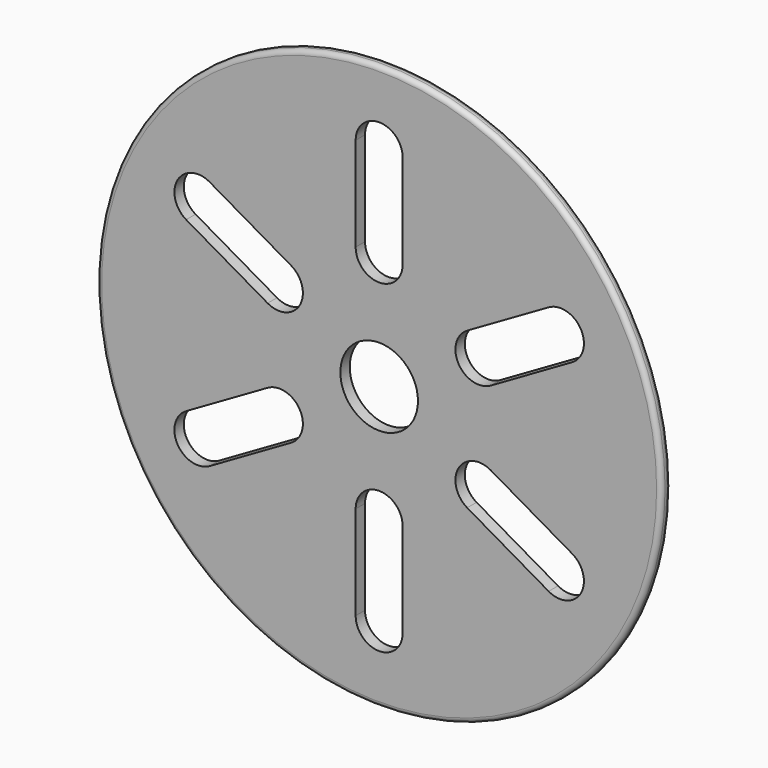
from build123d import *

# Parameters (mm, degrees)
F0_R     = 304.8
F0_R_2   = 41.91
F1_DEPTH = 12.7
F3_DEPTH = 12.701
F4_R     = 5.08


# Not quite as in the source:
# - a feature names something its author has since deleted; it is built from what else it names


with BuildPart() as f1:
    # F0 (on Front) → F1 (new body)
    with BuildSketch(Plane.XZ):
        Circle(F0_R)
        Circle(F0_R_2, mode=Mode.SUBTRACT)
    extrude(amount=F1_DEPTH)

    # F2 (on face) → F3 (cut, through all)
    with BuildSketch(Plane.XZ.offset(12.7)):
        with BuildLine():
            Line((-25.4, 226.06), (-25.4, 124.46))
            ThreePointArc((-25.4, 124.46), (0, 99.06), (25.4, 124.46))
            Line((25.4, 124.46), (25.4, 226.06))
            ThreePointArc((25.4, 226.06), (0, 251.46), (-25.4, 226.06))
        make_face()
        with BuildLine():
            Line((-183.0737027795, -135.0270452561), (-95.085521755, -84.2270452561))
            ThreePointArc((-95.085521755, -84.2270452561), (-85.7884764989, -49.53), (-120.485521755, -40.2329547439))
            Line((-120.485521755, -40.2329547439), (-208.4737027795, -91.0329547439))
            ThreePointArc((-208.4737027795, -91.0329547439), (-217.7707480356, -125.73), (-183.0737027795, -135.0270452561))
        make_face()
        with BuildLine():
            Line((-208.4737027795, 91.0329547439), (-120.485521755, 40.2329547439))
            ThreePointArc((-120.485521755, 40.2329547439), (-85.7884764989, 49.53), (-95.085521755, 84.2270452561))
            Line((-95.085521755, 84.2270452561), (-183.0737027795, 135.0270452561))
            ThreePointArc((-183.0737027795, 135.0270452561), (-217.7707480356, 125.73), (-208.4737027795, 91.0329547439))
        make_face()
        with BuildLine():
            Line((183.0737027795, 135.0270452561), (95.085521755, 84.2270452561))
            ThreePointArc((95.085521755, 84.2270452561), (85.7884764989, 49.53), (120.485521755, 40.2329547439))
            Line((120.485521755, 40.2329547439), (208.4737027795, 91.0329547439))
            ThreePointArc((208.4737027795, 91.0329547439), (217.7707480356, 125.73), (183.0737027795, 135.0270452561))
        make_face()
        with BuildLine():
            Line((208.4737027795, -91.0329547439), (120.485521755, -40.2329547439))
            ThreePointArc((120.485521755, -40.2329547439), (85.7884764989, -49.53), (95.085521755, -84.2270452561))
            Line((95.085521755, -84.2270452561), (183.0737027795, -135.0270452561))
            ThreePointArc((183.0737027795, -135.0270452561), (217.7707480356, -125.73), (208.4737027795, -91.0329547439))
        make_face()
        with BuildLine():
            Line((25.4, -226.06), (25.4, -124.46))
            ThreePointArc((25.4, -124.46), (0, -99.06), (-25.4, -124.46))
            Line((-25.4, -124.46), (-25.4, -226.06))
            ThreePointArc((-25.4, -226.06), (0, -251.46), (25.4, -226.06))
        make_face()
    extrude(amount=-F3_DEPTH, mode=Mode.SUBTRACT)

    # F4
    f4_edges = [f1.edges().sort_by_distance(p)[0] for p in [
        (-304.8, 0, 0),
        (-304.8, -12.7, 0),
    ]]
    fillet(f4_edges, radius=F4_R)


solid = f1.part
